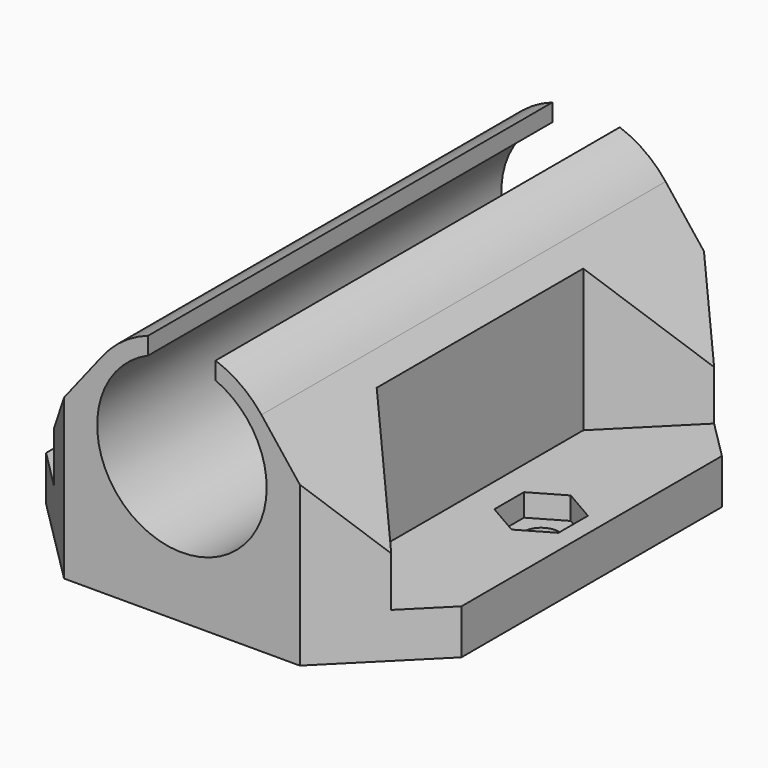
from build123d import *

# Parameters (mm, degrees)
F1_DEPTH    = 22.5
F3_W        = 9.95
F3_H        = 39
F4_DEPTH    = 12.6836794258
F5_R        = 1.55
F6_DEPTH    = 4
F7_DEPTH    = 2
F8_SIZE2    = 8
F8_SIZE     = 8
F9_T1_DEPTH = 45.1469278075


# Not quite as in the source:
# - a fillet or chamfer that OpenCascade refuses, or shapes differently, is made with other operations: its cross-section is extruded or revolved along the edge and cut away or added


with BuildPart() as f1:
    # F0 (on Front) → F1 (new body, symmetric)
    with BuildSketch(Plane.XZ):
        with BuildLine():
            Line((18.5, 4), (7.0809214412, 18.555227407))
            ThreePointArc((7.0809214412, 18.555227407), (8.5067118492, 15.9386822752), (9, 13))
            ThreePointArc((9, 13), (-2.9386822752, 4.4932881508), (-7.0809214412, 18.555227407))
            Line((-7.0809214412, 18.555227407), (-18.5, 4))
            Line((-18.5, 4), (-18.5, 0))
            Line((-18.5, 0), (18.5, 0))
            Line((18.5, 0), (18.5, 4))
        make_face()
        with BuildLine():
            ThreePointArc((3, 19.9283836499), (6.3108042277, 17.1444239648), (7.55, 13))
            ThreePointArc((7.55, 13), (-4.1444239648, 6.6891957723), (-3, 19.9283836499))
            Line((-3, 19.9283836499), (-3, 21.4852813742))
            ThreePointArc((-3, 21.4852813742), (-5.2490521372, 20.3107764062), (-7.0809214412, 18.555227407))
            ThreePointArc((-7.0809214412, 18.555227407), (-2.9386822752, 4.4932881508), (9, 13))
            ThreePointArc((9, 13), (8.5067118492, 15.9386822752), (7.0809214412, 18.555227407))
            ThreePointArc((7.0809214412, 18.555227407), (5.2490521372, 20.3107764062), (3, 21.4852813742))
            Line((3, 21.4852813742), (3, 19.9283836499))
        make_face()
    extrude(amount=F1_DEPTH, both=True)

    # F3 (on offset) → F4 (cut, through all)
    with BuildSketch(Plane.XY.offset(4)):
        with Locations((-13.525, 0)):
            Rectangle(F3_W, F3_H)
        with Locations((13.525, 0)):
            Rectangle(F3_W, F3_H)
    extrude(amount=F4_DEPTH, mode=Mode.SUBTRACT)

    # F5 (on face) → F6 (cut, through all)
    with BuildSketch(Plane.XY.offset(4)):
        with Locations((14, 0)):
            Circle(F5_R)
        with Locations((-14, 0)):
            Circle(F5_R)
    extrude(amount=-F6_DEPTH, mode=Mode.SUBTRACT)

    # F5 (on face) → F7 (cut)
    with BuildSketch(Plane.XY.offset(4)):
        Polygon((11.15, 1.6454482672), (11.15, -1.6454482672), (14, -3.2908965344), (16.85, -1.6454482672), (16.85, 1.6454482672), (14, 3.2908965344), align=None)
        with Locations((14, 0)):
            Circle(F5_R, mode=Mode.SUBTRACT)
        Polygon((-11.15, -1.6454482672), (-11.15, 1.6454482672), (-14, 3.2908965344), (-16.85, 1.6454482672), (-16.85, -1.6454482672), (-14, -3.2908965344), align=None)
        with Locations((-14, 0)):
            Circle(F5_R, mode=Mode.SUBTRACT)
    extrude(amount=-F7_DEPTH, mode=Mode.SUBTRACT)

    # F8
    f8_edges = [f1.edges().sort_by_distance(p)[0] for p in [
        (-8.55, 19.5, 10.34134),
        (-8.55, -19.5, 10.34134),
        (8.55, 19.5, 10.34134),
        (8.55, -19.5, 10.34134),
    ]]
    chamfer(f8_edges, length=F8_SIZE, length2=F8_SIZE2)

    # F9: chamfer of 8 on 4 edges, made by hand

    # F9_s2 → F9_t1 (cut)
    with BuildSketch(Plane.XY.offset(-20.5734639037)):
        Polygon((-10.5, 22.5), (-18.5, 14.5), (-18.5, 22.5), align=None)
        Polygon((-10.5, -22.5), (-18.5, -14.5), (-18.5, -22.5), align=None)
        Polygon((18.5, 14.5), (10.5, 22.5), (18.5, 22.5), align=None)
        Polygon((18.5, -14.5), (10.5, -22.5), (18.5, -22.5), align=None)
    extrude(amount=F9_T1_DEPTH, mode=Mode.SUBTRACT)


solid = f1.part
